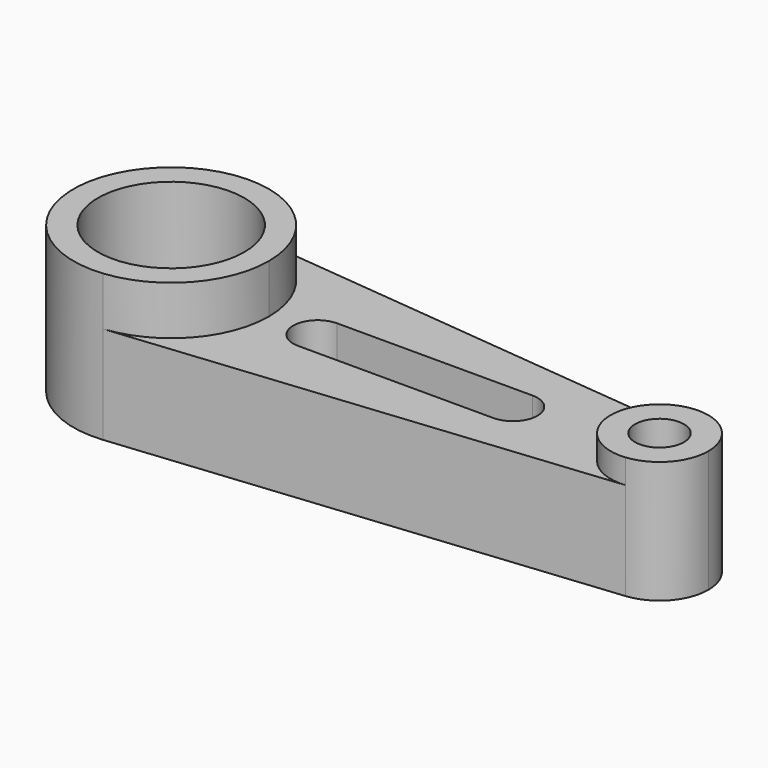
from build123d import *
from build123d import SkipClean  # not in build123d's __all__

# Parameters (mm, degrees)
F0_R     = 19.05
F0_R_2   = 6.35
F1_DEPTH = 38.1
F2_DEPTH = 12.7
F3_DEPTH = 6.35


with BuildPart() as f1:
    # F0 (on Top) → F1 (new body)
    with BuildSketch(Plane.XY):
        with BuildLine():
            ThreePointArc((-35.56, -25.2726809025), (-19.2628558428, -17.0388379885), (-12.7, 0))
            ThreePointArc((-12.7, 0), (-19.2628558428, 17.0388379885), (-35.56, 25.2726809025))
            ThreePointArc((-35.56, 25.2726809025), (-63.5, 0), (-35.56, -25.2726809025))
        make_face()
        with Locations((-38.1, 0)):
            Circle(F0_R, mode=Mode.SUBTRACT)
        with BuildLine():
            ThreePointArc((-35.56, 25.2726809025), (-19.2628558428, 17.0388379885), (-12.7, 0))
            ThreePointArc((-12.7, 0), (-19.2628558428, -17.0388379885), (-35.56, -25.2726809025))
            Line((-35.56, -25.2726809025), (90.17, -12.6363404513))
            ThreePointArc((90.17, -12.6363404513), (76.2, 0), (90.17, 12.6363404513))
            Line((90.17, 12.6363404513), (-35.56, 25.2726809025))
        make_face()
        with BuildLine():
            ThreePointArc((0, -6.35), (-6.35, 0), (0, 6.35))
            Line((0, 6.35), (50.8, 6.35))
            ThreePointArc((50.8, 6.35), (55.2901280605, 4.4901280605), (57.15, 0))
            ThreePointArc((57.15, 0), (55.2901280605, -4.4901280605), (50.8, -6.35))
            Line((50.8, -6.35), (0, -6.35))
        make_face(mode=Mode.SUBTRACT)
        with BuildLine():
            ThreePointArc((101.6, 0), (98.3185720786, 8.5194189943), (90.17, 12.6363404513))
            ThreePointArc((90.17, 12.6363404513), (76.2, 0), (90.17, -12.6363404513))
            ThreePointArc((90.17, -12.6363404513), (98.3185720786, -8.5194189943), (101.6, 0))
        make_face()
        with Locations((88.9, 0)):
            Circle(F0_R_2, mode=Mode.SUBTRACT)
    extrude(amount=-F1_DEPTH)

    # F0 (on Top) → F2 (cut)
    with BuildSketch(Plane.XY):
        with BuildLine():
            ThreePointArc((-35.56, 25.2726809025), (-19.2628558428, 17.0388379885), (-12.7, 0))
            ThreePointArc((-12.7, 0), (-19.2628558428, -17.0388379885), (-35.56, -25.2726809025))
            Line((-35.56, -25.2726809025), (90.17, -12.6363404513))
            ThreePointArc((90.17, -12.6363404513), (76.2, 0), (90.17, 12.6363404513))
            Line((90.17, 12.6363404513), (-35.56, 25.2726809025))
        make_face()
        with BuildLine():
            ThreePointArc((0, -6.35), (-6.35, 0), (0, 6.35))
            Line((0, 6.35), (50.8, 6.35))
            ThreePointArc((50.8, 6.35), (55.2901280605, 4.4901280605), (57.15, 0))
            ThreePointArc((57.15, 0), (55.2901280605, -4.4901280605), (50.8, -6.35))
            Line((50.8, -6.35), (0, -6.35))
        make_face(mode=Mode.SUBTRACT)
    with SkipClean():  # cleaning this boolean's faces spoils the solid; the shape is the same uncleaned
        extrude(amount=-F2_DEPTH, mode=Mode.SUBTRACT)

    # F0 (on Top) → F3 (cut)
    with BuildSketch(Plane.XY):
        with BuildLine():
            ThreePointArc((101.6, 0), (98.3185720786, 8.5194189943), (90.17, 12.6363404513))
            ThreePointArc((90.17, 12.6363404513), (76.2, 0), (90.17, -12.6363404513))
            ThreePointArc((90.17, -12.6363404513), (98.3185720786, -8.5194189943), (101.6, 0))
        make_face()
        with Locations((88.9, 0)):
            Circle(F0_R_2, mode=Mode.SUBTRACT)
    extrude(amount=-F3_DEPTH, mode=Mode.SUBTRACT)


solid = f1.part
